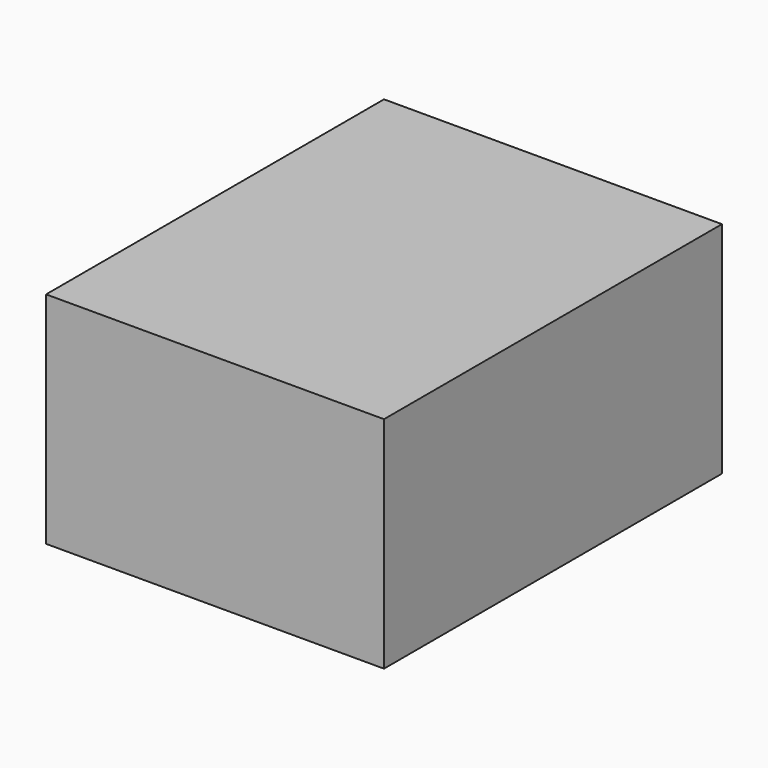
from build123d import *

# Parameters (mm, degrees)
F0_W           = 50.8
F0_H           = 63.5
F1_DEPTH       = 7.62
F2_W           = 50.8
F2_H           = 63.5
F3_W           = 50.8
F3_H           = 63.5
F3_TEXT_SIZE   = 17.046560404
F3_TEXT_SIZE_2 = 17.8453816463
F1_FACE_W      = 50.8
F1_FACE_H      = 63.5
F1_FACE1_W     = 50.8
F1_FACE1_H     = 63.5
F4_DEPTH       = 25.4


# Not quite as in the source:
# - Text() gives the source's letters only with a copy of the font that has no kerning and outlines rounded to 1/6400 em; it was checked with that copy


with BuildPart() as f1:
    # F0 (on Top) → F1 (new body)
    with BuildSketch(Plane.XY):
        with Locations((31.1732371277, 31.75)):
            Rectangle(F0_W, F0_H)
    extrude(amount=F1_DEPTH)

    # F2 (on face) + F3 (on face) + F1_face (on face) + F1_face1 (on face) → F4 (join)
    with BuildSketch(Plane.XY.offset(7.62)):
        with Locations((31.1732371277, 31.75)):
            Rectangle(F2_W, F2_H)
    with BuildSketch(Plane.XY.offset(7.62)):
        with Locations((31.1732371277, 31.75)):
            Rectangle(F3_W, F3_H)
        Polygon((24.1447914516, 3.8936187048), (23.6484667745, 7.9450780066), (19.3265384071, 7.9450780066), (17.1906692913, 3.8936187048), (15.5427598299, 3.8936187048), (22.5052470128, 16.6335481957), (24.0221044527, 16.6335481957), (25.62540046, 3.8936187048), align=None, mode=Mode.SUBTRACT)
        with BuildLine():
            Line((36.0014248334, 4.4687699992), (34.8614361063, 4.4687699992))
            Line((34.8614361063, 4.4687699992), (30.7329722585, 15.2560465049))
            Line((30.7329722585, 15.2560465049), (30.6663841319, 15.2560465049))
            add(Edge.make_bspline(
                [(30.6663841319, 15.2560465049), (30.7835792347, 13.9748909495), (30.7835792347, 12.2089738327)],
                knots=[0, 0, 0, 1, 1, 1], degree=2))
            Line((30.7835792347, 12.2089738327), (30.7835792347, 4.4687699992))
            Line((30.7835792347, 4.4687699992), (29.4757884287, 4.4687699992))
            Line((29.4757884287, 4.4687699992), (29.4757884287, 16.6384160126))
            Line((29.4757884287, 16.6384160126), (31.6066084792, 16.6384160126))
            Line((31.6066084792, 16.6384160126), (35.4607292455, 6.5995900497))
            Line((35.4607292455, 6.5995900497), (35.5273173721, 6.5995900497))
            Line((35.5273173721, 6.5995900497), (39.4134004392, 16.6384160126))
            Line((39.4134004392, 16.6384160126), (41.5282393393, 16.6384160126))
            Line((41.5282393393, 16.6384160126), (41.5282393393, 4.4687699992))
            Line((41.5282393393, 4.4687699992), (40.1139075308, 4.4687699992))
            Line((40.1139075308, 4.4687699992), (40.1139075308, 12.3101877851))
            add(Edge.make_bspline(
                [(40.1139075308, 12.3101877851), (40.1139075308, 13.657931467), (40.2311026336, 15.2400653545)],
                knots=[0, 0, 0, 1, 1, 1], degree=2))
            Line((40.2311026336, 15.2400653545), (40.164514507, 15.2400653545))
            Line((40.164514507, 15.2400653545), (36.0014248334, 4.4687699992))
        make_face(mode=Mode.SUBTRACT)
        with BuildLine():
            add(Edge.make_bspline(
                [(47.46257318, 16.6384160126), (52.022528088, 16.6384160126), (52.022528088, 13.0932641536)],
                knots=[0, 0, 0, 1, 1, 1], degree=2))
            add(Edge.make_bspline(
                [(52.022528088, 13.0932641536), (52.022528088, 11.2447777598), (50.7613489707, 10.2499511487)],
                knots=[0, 0, 0, 1, 1, 1], degree=2))
            add(Edge.make_bspline(
                [(50.7613489707, 10.2499511487), (49.5001698533, 9.2551245377), (47.1536042727, 9.2551245377)],
                knots=[0, 0, 0, 1, 1, 1], degree=2))
            Line((47.1536042727, 9.2551245377), (45.7206277887, 9.2551245377))
            Line((45.7206277887, 9.2551245377), (45.7206277887, 4.4687699992))
            Line((45.7206277887, 4.4687699992), (44.3062959802, 4.4687699992))
            Line((44.3062959802, 4.4687699992), (44.3062959802, 16.6384160126))
            Line((44.3062959802, 16.6384160126), (47.46257318, 16.6384160126))
        make_face(mode=Mode.SUBTRACT)
        with Locations((27.8030946891, 4.4687699992)):
            Text('M', F3_TEXT_SIZE, font='Open Sans', text_align=(TextAlign.LEFT, TextAlign.BOTTOM))
        with Locations((42.6336022405, 4.4687699992)):
            Text('P', F3_TEXT_SIZE, font='Open Sans', text_align=(TextAlign.LEFT, TextAlign.BOTTOM))
        with Locations((16.5632925928, 3.8936187048)):
            Text('A', F3_TEXT_SIZE_2, font='Open Sans', font_style=FontStyle.ITALIC, text_align=(TextAlign.LEFT, TextAlign.BOTTOM))
        with BuildLine():
            Line((20.0570837182, 9.3057883572), (23.4895313442, 9.3057883572))
            Line((23.4895313442, 9.3057883572), (23.1856021881, 11.9100987412))
            add(Edge.make_bspline(
                [(23.1856021881, 11.9100987412), (22.9764766219, 13.4687812944), (22.9318631678, 14.9605436663)],
                knots=[0, 0, 0, 1, 1, 1], degree=2))
            add(Edge.make_bspline(
                [(22.9318631678, 14.9605436663), (22.6112039663, 14.1937499237), (22.2319896064, 13.4353212038)],
                knots=[0, 0, 0, 1, 1, 1], degree=2))
            add(Edge.make_bspline(
                [(22.2319896064, 13.4353212038), (21.8527752464, 12.6768924838), (20.0570837182, 9.3057883572)],
                knots=[0, 0, 0, 1, 1, 1], degree=2))
        make_face()
    with BuildSketch(Plane(origin=(31.1732371277, 31.75, 7.62), x_dir=(1, 0, 0), z_dir=(0, 0, 1))):
        Rectangle(F1_FACE_W, F1_FACE_H)
    with BuildSketch(Plane(origin=(31.1732371277, 31.75, 0), x_dir=(1, 0, 0), z_dir=(0, 0, -1))):
        Rectangle(F1_FACE1_W, F1_FACE1_H)
    extrude(amount=-F4_DEPTH, dir=(0, 0, 1))


solid = f1.part
